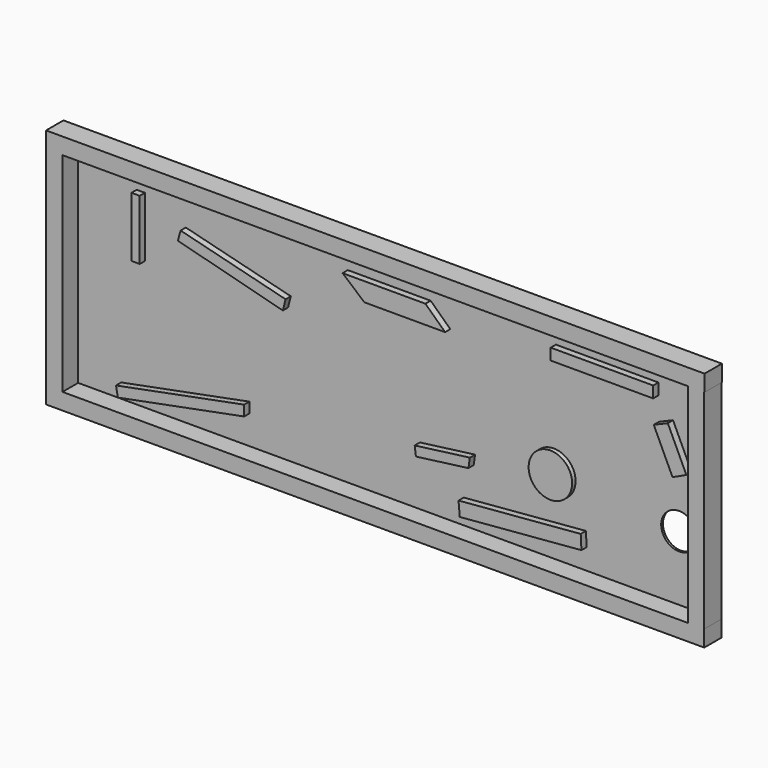
from build123d import *

# Parameters (mm, degrees)
F1_DEPTH = 63.5
F0_R     = 63.6308259599
F0_R_2   = 52.2581940634
F0_W     = 24.2178440094
F0_H     = 175.5797639489
F0_W_2   = 299.6964156628
F0_H_2   = 33.2996025681
F2_DEPTH = 6.35
F5_DEPTH = 25.4
F6_DEPTH = 19.05


# Not quite as in the source:
# - the program builds the solid bodies; features that only make, move or delete a surface that nothing else refers to are left out


with BuildPart() as f1:
    # F0 (on Front) → F1 (new body)
    with BuildSketch(Plane.XZ):
        Polygon((-969.1663980484, 198.6485360199), (-921.1349980484, 198.6485360199), (907.6650019516, 198.6485360199), (955.6964019516, 198.6485360199), (956.6172361374, 198.6485360199), (956.6172361374, 246.6799360199), (-969.1663980484, 246.6799360199), align=None)
        Polygon((-921.1349980484, -371.5092837811), (-921.1349980484, 198.6485360199), (-969.1663980484, 198.6485360199), (-969.1663980484, -410.9517233025), (-921.1349980484, -410.9517233025), (-921.1349980484, -410.9514639801), align=None)
        Polygon((-921.1349980484, -410.9517233025), (-969.1663980484, -410.9517233025), (-969.1663980484, -458.9831233025), (955.726981163, -458.9831233025), (955.726981163, -410.9517233025), (955.6964019516, -410.9517233025), (907.6650019516, -410.9517233025), align=None)
        Polygon((955.6964019516, 198.6485360199), (907.6650019516, 198.6485360199), (907.6650019516, -410.9514639801), (907.6650019516, -410.9517233025), (955.6964019516, -410.9517233025), align=None)
    extrude(amount=F1_DEPTH)

    # F0 (on Front) → F2 (join)
    with BuildSketch(Plane.XZ):
        Polygon((907.6650019516, 198.6485360199), (-921.1349980484, 198.6485360199), (-921.1349980484, -371.5092837811), (-921.1349980484, -410.9514639801), (-31.4717553556, -410.9514639801), (907.6650019516, -410.9514639801), align=None)
        Polygon((-789.5849161051, -398.2566583191), (-795.2640652657, -368.8750267029), (-420.4561412334, -296.4287400246), (-420.4561412334, -326.9080892764), align=None, mode=Mode.SUBTRACT)
        Polygon((210.169616585, -380.4944990589), (206.6856175661, -339.3833041191), (563.899576664, -309.1109395027), (566.059074651, -350.3343802749), align=None, mode=Mode.SUBTRACT)
        Polygon((235.5920225382, -246.5991973877), (81.9196328521, -266.643434763), (78.3429656397, -239.222336751), (239.8227507102, -218.1597428141), align=None, mode=Mode.SUBTRACT)
        with Locations((470.1542854309, -190.9026801586)):
            Circle(F0_R, mode=Mode.SUBTRACT)
        with Locations((836.3508582115, -221.3210761547)):
            Circle(F0_R_2, mode=Mode.SUBTRACT)
        with Locations((-737.8122806549, 54.1574768722)):
            Rectangle(F0_W, F0_H, mode=Mode.SUBTRACT)
        Polygon((-614.0667200089, 62.5602602959), (-606.2821745872, 91.4887040854), (-299.1916835308, 14.3223749474), (-307.1056894279, -17.1721380653), align=None, mode=Mode.SUBTRACT)
        Polygon((777.5867510857, 41.2790888272), (818.6616301537, 58.8090009987), (872.9156851768, -56.7944645882), (832.5127084301, -75.7560529142), align=None, mode=Mode.SUBTRACT)
        Polygon((-132.3649287224, 135.8928531408), (109.8140254617, 135.8928531408), (167.3315316439, 81.402592361), (-68.7929466367, 81.402592361), align=None, mode=Mode.SUBTRACT)
        with Locations((625.9579211473, 125.2975575626)):
            Rectangle(F0_W_2, F0_H_2, mode=Mode.SUBTRACT)
        Polygon((907.6650019516, -410.9517233025), (907.6650019516, -410.9514639801), (-31.4717553556, -410.9514639801), (-921.1349980484, -410.9514639801), (-921.1349980484, -410.9517233025), align=None)
    extrude(amount=F2_DEPTH)

    # F0 (on Front) → F5 (join)
    with BuildSketch(Plane.XZ):
        with Locations((625.9579211473, 125.2975575626)):
            Rectangle(F0_W_2, F0_H_2)
        Polygon((167.3315316439, 81.402592361), (109.8140254617, 135.8928531408), (-132.3649287224, 135.8928531408), (-68.7929466367, 81.402592361), align=None)
        Polygon((-299.1916835308, 14.3223749474), (-606.2821745872, 91.4887040854), (-614.0667200089, 62.5602602959), (-307.1056894279, -17.1721380653), align=None)
        Polygon((-420.4561412334, -296.4287400246), (-795.2640652657, -368.8750267029), (-789.5849161051, -398.2566583191), (-420.4561412334, -326.9080892764), align=None)
        Polygon((78.3429656397, -239.222336751), (81.9196328521, -266.643434763), (235.5920225382, -246.5991973877), (239.8227507102, -218.1597428141), align=None)
        Polygon((563.899576664, -309.1109395027), (206.6856175661, -339.3833041191), (210.169616585, -380.4944990589), (566.059074651, -350.3343802749), align=None)
        with Locations((-737.8122806549, 54.1574768722)):
            Rectangle(F0_W, F0_H)
        Polygon((872.9156851768, -56.7944645882), (818.6616301537, 58.8090009987), (777.5867510857, 41.2790888272), (832.5127084301, -75.7560529142), align=None)
    extrude(amount=F5_DEPTH)

    # F0 (on Front) → F6 (join)
    with BuildSketch(Plane.XZ):
        with Locations((470.1542854309, -190.9026801586)):
            Circle(F0_R)
    extrude(amount=F6_DEPTH)


solid = f1.part
